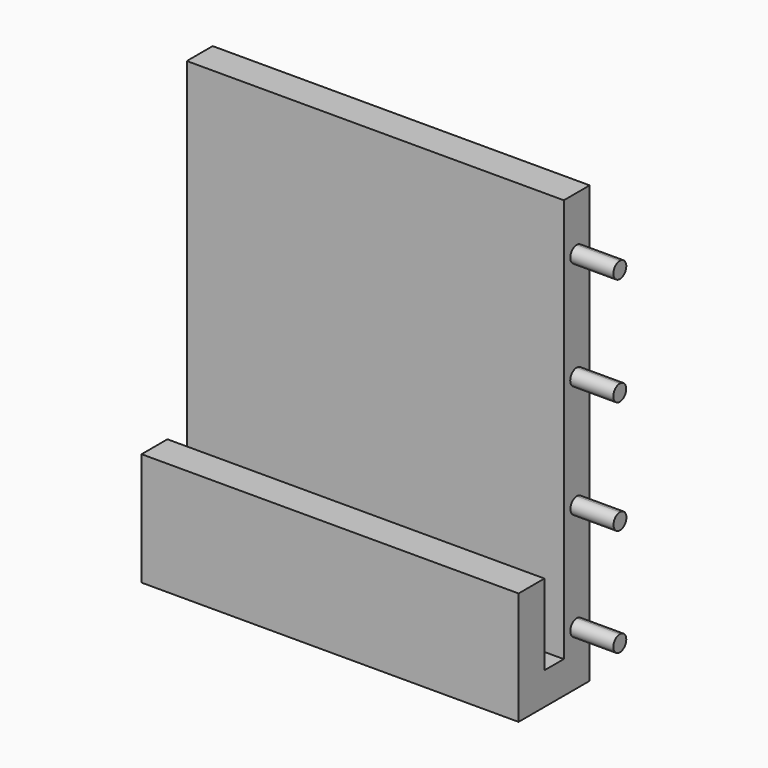
from build123d import *

# Parameters (mm, degrees)
F1_DEPTH = 70
F3_DEPTH = 8
F5_DEPTH = 9
F6_R     = 1.875
F7_DEPTH = 9


# Not quite as in the source:
# - a feature names something its author has since deleted; it is built from what else it names


with BuildPart() as f1:
    # F0 (on Right) → F1 (new body)
    with BuildSketch(Plane.YZ):
        Polygon((15.9777059274, -37.1211464703), (15.9777059274, 43.8788535297), (9.9777059274, 43.8788535297), (9.9777059274, -31.1211464703), (5.4777059274, -31.1211464703), (5.4777059274, -16.1211464703), (-0.5222940726, -16.1211464703), (-0.5222940726, -37.1211464703), align=None)
    extrude(amount=F1_DEPTH)

    # F2 (on face) → F3 (join)
    with BuildSketch(Plane.YZ.offset(70)):
        with BuildLine():
            Line((12.9777059274, 33.8788535297), (12.9777059274, 35.3788535297))
            ThreePointArc((12.9777059274, 35.3788535297), (11.4777059274, 33.8788535297), (12.9777059274, 32.3788535297))
            Line((12.9777059274, 32.3788535297), (12.9777059274, 33.8788535297))
        make_face()
        with BuildLine():
            ThreePointArc((12.9777059274, 32.3788535297), (14.0383660992, 32.8181933579), (14.4777059274, 33.8788535297))
            ThreePointArc((14.4777059274, 33.8788535297), (14.0383660992, 34.9395137015), (12.9777059274, 35.3788535297))
            Line((12.9777059274, 35.3788535297), (12.9777059274, 33.8788535297))
            Line((12.9777059274, 33.8788535297), (12.9777059274, 32.3788535297))
        make_face()
        with BuildLine():
            Line((12.9777059274, 13.8788535297), (12.9777059274, 15.3178830066))
            ThreePointArc((12.9777059274, 15.3178830066), (11.4636811456, 13.8179485729), (12.9777059274, 12.3180141391))
            Line((12.9777059274, 12.3180141391), (12.9777059274, 13.8788535297))
        make_face()
        with BuildLine():
            ThreePointArc((14.4636811456, 13.8179485729), (14.0292882901, 14.8736385906), (12.9777059274, 15.3178830066))
            Line((12.9777059274, 15.3178830066), (12.9777059274, 13.8788535297))
            Line((12.9777059274, 13.8788535297), (12.9777059274, 12.3180141391))
            ThreePointArc((12.9777059274, 12.3180141391), (14.0292882901, 12.7622585551), (14.4636811456, 13.8179485729))
        make_face()
        with BuildLine():
            Line((12.9777059274, -7.1211464703), (12.9777059274, -5.7047228841))
            ThreePointArc((12.9777059274, -5.7047228841), (11.5072213267, -7.2044324698), (12.9777059274, -8.7041420554))
            Line((12.9777059274, -8.7041420554), (12.9777059274, -7.1211464703))
        make_face()
        with BuildLine():
            ThreePointArc((14.5072213267, -7.2044324698), (14.0573943841, -6.1333878631), (12.9777059274, -5.7047228841))
            Line((12.9777059274, -5.7047228841), (12.9777059274, -7.1211464703))
            Line((12.9777059274, -7.1211464703), (12.9777059274, -8.7041420554))
            ThreePointArc((12.9777059274, -8.7041420554), (14.0573943841, -8.2754770764), (14.5072213267, -7.2044324698))
        make_face()
        with BuildLine():
            ThreePointArc((12.9777059274, -25.6469734003), (11.473965778, -27.1469687374), (12.9777059274, -28.6469640745))
            Line((12.9777059274, -28.6469640745), (12.9777059274, -27.1211464703))
            Line((12.9777059274, -27.1211464703), (12.9777059274, -25.6469734003))
        make_face()
        with BuildLine():
            Line((12.9777059274, -27.1211464703), (12.9777059274, -28.6469640745))
            ThreePointArc((12.9777059274, -28.6469640745), (14.035947469, -28.2063057413), (14.473965778, -27.1469687374))
            ThreePointArc((14.473965778, -27.1469687374), (14.035947469, -26.0876317334), (12.9777059274, -25.6469734003))
            Line((12.9777059274, -25.6469734003), (12.9777059274, -27.1211464703))
        make_face()
    extrude(amount=F3_DEPTH)

    # F4 (on face) → F5 (cut)
    with BuildSketch(Plane(origin=(0, 0, 0), x_dir=(0, -1, 0), z_dir=(-1, 0, 0))):
        with BuildLine():
            ThreePointArc((-12.9777059274, 32.0038535297), (-11.6518807127, 32.553028315), (-11.1027059274, 33.8788535297))
            ThreePointArc((-11.1027059274, 33.8788535297), (-11.6518807127, 35.2046787444), (-12.9777059274, 35.7538535297))
            Line((-12.9777059274, 35.7538535297), (-12.9777059274, 33.8788535297))
            Line((-12.9777059274, 33.8788535297), (-12.9777059274, 32.0038535297))
        make_face()
        with BuildLine():
            Line((-12.9777059274, 33.8788535297), (-12.9777059274, 35.7538535297))
            ThreePointArc((-12.9777059274, 35.7538535297), (-14.8527059274, 33.8788535297), (-12.9777059274, 32.0038535297))
            Line((-12.9777059274, 32.0038535297), (-12.9777059274, 33.8788535297))
        make_face()
        with BuildLine():
            ThreePointArc((-11.1027059274, 13.8788535297), (-11.6518807127, 15.2046787444), (-12.9777059274, 15.7538535297))
            ThreePointArc((-12.9777059274, 15.7538535297), (-14.3035311422, 12.553028315), (-11.1027059274, 13.8788535297))
        make_face()
        with BuildLine():
            ThreePointArc((-11.1027059274, -7.1211464703), (-14.3035311422, -5.7953212556), (-12.9777059274, -8.9961464703))
            ThreePointArc((-12.9777059274, -8.9961464703), (-11.6518807127, -8.446971685), (-11.1027059274, -7.1211464703))
        make_face()
        with BuildLine():
            ThreePointArc((-12.9777059274, -25.2461464703), (-14.8527059274, -27.1211464703), (-12.9777059274, -28.9961464703))
            Line((-12.9777059274, -28.9961464703), (-12.9777059274, -27.1211464703))
            Line((-12.9777059274, -27.1211464703), (-12.9777059274, -25.2461464703))
        make_face()
        with BuildLine():
            Line((-12.9777059274, -27.1211464703), (-12.9777059274, -28.9961464703))
            ThreePointArc((-12.9777059274, -28.9961464703), (-11.6518807127, -28.446971685), (-11.1027059274, -27.1211464703))
            ThreePointArc((-11.1027059274, -27.1211464703), (-11.6518807127, -25.7953212556), (-12.9777059274, -25.2461464703))
            Line((-12.9777059274, -25.2461464703), (-12.9777059274, -27.1211464703))
        make_face()
    extrude(amount=-F5_DEPTH, mode=Mode.SUBTRACT)

    # F6 (on face) → F7 (cut)
    with BuildSketch(Plane(origin=(0, 15.9777059274, 0), x_dir=(-1, 0, 0), z_dir=(0, 1, 0))):
        with Locations((-55, -34.1211464703)):
            Circle(F6_R)
        with Locations((-35, -34.1211464703)):
            Circle(F6_R)
        with Locations((-15, -34.1211464703)):
            Circle(F6_R)
    extrude(amount=-F7_DEPTH, mode=Mode.SUBTRACT)


solid = f1.part
